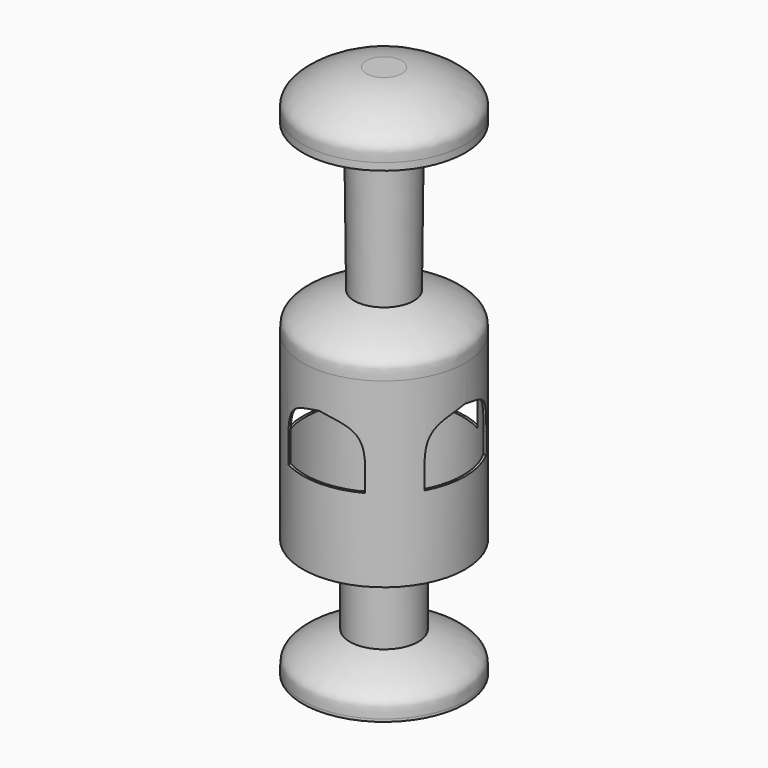
from build123d import *

# Parameters (mm, degrees)
F4_DEPTH = 25
F6_DEPTH = 25


# Not quite as in the source:
# - the dataset's text gives a spline's control points without its knots; the knots are read off the source's solid


with BuildPart() as f1:
    # F0 (on Front) → F1 (revolve)
    with BuildSketch(Plane.XZ):
        with BuildLine():
            Line((20.2840724203, -27.343348276), (23.0495763149, -27.3330021896))
            Line((23.0495763149, -27.3330021896), (23.0495763149, 24.1761978883))
            add(Edge.make_bspline(
                [(23.0495763149, 24.1761978883), (22.8941435237, 26.0308608144), (23.9395420726, 29.003648868), (14.0261189654, 33.6296849109), (8.4189805979, 34.9379997258)],
                knots=[0, 0, 0, 0, 0.3260886129, 0.8771804513, 0.8771804513, 0.8771804513, 0.8771804513], degree=3))
            add(Edge.make_bspline(
                [(8.4189805979, 34.9379997258), (8.1849872822, 34.992597437), (7.9520754508, 35.0444122094), (7.7206045906, 35.0932804837)],
                knots=[0.8771804513, 0.8771804513, 0.8771804513, 0.8771804513, 0.9001782441, 0.9001782441, 0.9001782441, 0.9001782441], degree=3))
            add(Edge.make_bspline(
                [(7.7206045906, 35.0932804837), (6.7159069707, 35.3053928798), (5.7383570717, 35.4619936087), (4.8173516989, 35.5497077107)],
                knots=[0.9001782441, 0.9001782441, 0.9001782441, 0.9001782441, 1, 1, 1, 1], degree=3))
            Line((4.8173516989, 35.5497077107), (0, 35.5497077107))
            Line((0, 35.5497077107), (0, 34.6961133182))
            Line((0, 34.6961133182), (4.8552267253, 34.6961133182))
            add(Edge.make_bspline(
                [(22.3495763149, 23.4555121765), (22.1897726726, 25.3623291907), (23.6752847702, 29.0289436305), (10.9884647614, 34.112000041), (4.8552267253, 34.6961133182)],
                knots=[0, 0, 0, 0, 0.3352583947, 1, 1, 1, 1], degree=3))
            Line((22.3495763149, 23.4555121765), (22.3495763149, -26.6947299242))
            Line((22.3495763149, -26.6947299242), (0, -26.6947299242))
            Line((0, -26.6947299242), (0, -27.4192334573))
            Line((0, -27.4192334573), (8.9649282769, -27.3856945706))
            Line((8.9649282769, -27.3856945706), (9.7, -27.3829445779))
            Line((9.7, -27.3829445779), (18.8340822147, -27.3487728656))
            Line((18.8340822147, -27.3487728656), (20.2840724203, -27.343348276))
        make_face()
    revolve(axis=Axis((0, 0, -7.0726890117), (0, 0, -1)))

    # F0 (on Front) → F2 (revolve)
    with BuildSketch(Plane.XZ):
        with BuildLine():
            add(Edge.make_bspline(
                [(23.0495763149, -60.2150011641), (22.8941435237, -58.3603382379), (23.8898585914, -55.5288345389), (14.9436544002, -51.1974927604), (9.7, -49.7765717533)],
                knots=[0, 0, 0, 0, 0.3260886129, 0.8354916825, 0.8354916825, 0.8354916825, 0.8354916825], degree=3))
            add(Edge.make_bspline(
                [(9.7, -49.7765717533), (9.4543795426, -49.7100137308), (9.2092217969, -49.6461323577), (8.9649282769, -49.5851103148)],
                knots=[0.8354916825, 0.8354916825, 0.8354916825, 0.8354916825, 0.8593528689, 0.8593528689, 0.8593528689, 0.8593528689], degree=3))
            add(Edge.make_bspline(
                [(8.9649282769, -49.5851103148), (7.5249670698, -49.2254226142), (6.1150323727, -48.9650789974), (4.8173516989, -48.8414913416)],
                knots=[0.8593528689, 0.8593528689, 0.8593528689, 0.8593528689, 1, 1, 1, 1], degree=3))
            Line((4.8173516989, -48.8414913416), (0, -48.8414913416))
            Line((0, -48.8414913416), (0, -49.6950857341))
            Line((0, -49.6950857341), (4.8552267253, -49.6950857341))
            add(Edge.make_bspline(
                [(22.3156850975, -60.2261610329), (22.2921596802, -58.7073440576), (23.1236631734, -55.1412446649), (10.9884647614, -50.2791990114), (4.8552267253, -49.6950857341)],
                knots=[0.0434798946, 0.0434798946, 0.0434798946, 0.0434798946, 0.3352583947, 1, 1, 1, 1], degree=3))
            add(Edge.make_bspline(
                [(22.3495763149, -60.9356868758), (22.3288512693, -60.6883904498), (22.3191907796, -60.4524902586), (22.3156850975, -60.2261610329)],
                knots=[0, 0, 0, 0, 0.0434798946, 0.0434798946, 0.0434798946, 0.0434798946], degree=3))
            Line((22.3495763149, -60.9356868758), (23.0495763149, -60.9422326088))
            Line((23.0495763149, -60.9422326088), (23.0495763149, -60.2150011641))
        make_face()
        with BuildLine():
            Line((9.7, -49.5851103148), (9.7, -27.3829445779))
            Line((9.7, -27.3829445779), (8.9649282769, -27.3856945706))
            Line((8.9649282769, -27.3856945706), (8.9649282769, -28.0694384128))
            Line((8.9649282769, -28.0694384128), (8.9649282769, -49.5851103148))
            add(Edge.make_bspline(
                [(9.7, -49.7765717533), (9.4543795426, -49.7100137308), (9.2092217969, -49.6461323577), (8.9649282769, -49.5851103148)],
                knots=[0.8354916825, 0.8354916825, 0.8354916825, 0.8354916825, 0.8593528689, 0.8593528689, 0.8593528689, 0.8593528689], degree=3))
            Line((9.7, -49.7765717533), (9.7, -49.5851103148))
        make_face()
        with BuildLine():
            Line((0, -60.9356868758), (22.3495763149, -60.9356868758))
            add(Edge.make_bspline(
                [(22.3495763149, -60.9356868758), (22.3288512693, -60.6883904498), (22.3191907796, -60.4524902586), (22.3156850975, -60.2261610329)],
                knots=[0, 0, 0, 0, 0.0434798946, 0.0434798946, 0.0434798946, 0.0434798946], degree=3))
            Line((22.3156850975, -60.2261610329), (0, -60.2261610329))
            Line((0, -60.2261610329), (0, -60.9356868758))
        make_face()
        Polygon((8.9649282769, -28.0694384128), (8.9649282769, -27.3856945706), (0, -27.4192334573), (0, -28.0694384128), align=None)
    revolve(axis=Axis((0, 0, -7.0726890117), (0, 0, -1)))

    # F3 (on Right) → F4 (cut, symmetric)
    with BuildSketch(Plane.YZ):
        with BuildLine():
            Line((-10.9680155292, -4.0999995545), (-0.0928910449, -4.0999995545))
            Line((-0.0928910449, -4.0999995545), (10.7822334394, -4.0999995545))
            Line((10.7822334394, -4.0999995545), (10.7822334394, 1.6936261673))
            add(Edge.make_bspline(
                [(10.7822334394, 1.6936261673), (10.8915483579, 10.6573491357), (8.377331309, 12.5156822614), (-0.0928910449, 14.0460734256)],
                knots=[0, 0, 0, 0, 16.4575601417, 16.4575601417, 16.4575601417, 16.4575601417], degree=3))
            add(Edge.make_bspline(
                [(-10.9680155292, 1.6936261673), (-11.0773304477, 10.6573491357), (-8.5631133988, 12.5156822614), (-0.0928910449, 14.0460734256)],
                knots=[0, 0, 0, 0, 16.4575601417, 16.4575601417, 16.4575601417, 16.4575601417], degree=3))
            Line((-10.9680155292, 1.6936261673), (-10.9680155292, -4.0999995545))
        make_face()
    extrude(amount=F4_DEPTH, both=True, mode=Mode.SUBTRACT)

    # F5 (on Front) → F6 (cut, symmetric)
    with BuildSketch(Plane.XZ):
        with BuildLine():
            Line((-10.8819976449, -3.9999997243), (-0.0068731606, -3.9999997243))
            Line((-0.0068731606, -3.9999997243), (10.8682513237, -3.9999997243))
            Line((10.8682513237, -3.9999997243), (10.8682513237, 1.7936259974))
            add(Edge.make_bspline(
                [(10.8682513237, 1.7936259974), (10.9775662422, 10.7573489659), (8.4633491933, 12.6156820916), (-0.0068731606, 14.1460732557)],
                knots=[0, 0, 0, 0, 16.4575601417, 16.4575601417, 16.4575601417, 16.4575601417], degree=3))
            add(Edge.make_bspline(
                [(-10.8819976449, 1.7936259974), (-10.9913125634, 10.7573489659), (-8.4770955145, 12.6156820916), (-0.0068731606, 14.1460732557)],
                knots=[0, 0, 0, 0, 16.4575601417, 16.4575601417, 16.4575601417, 16.4575601417], degree=3))
            Line((-10.8819976449, 1.7936259974), (-10.8819976449, -3.9999997243))
        make_face()
    extrude(amount=F6_DEPTH, both=True, mode=Mode.SUBTRACT)

    # F0 (on Front) → F7 (revolve)
    with BuildSketch(Plane.XZ):
        with BuildLine():
            add(Edge.make_bspline(
                [(8.4189805979, 34.9379997258), (8.1849872822, 34.992597437), (7.9520754508, 35.0444122094), (7.7206045906, 35.0932804837)],
                knots=[0.8771804513, 0.8771804513, 0.8771804513, 0.8771804513, 0.9001782441, 0.9001782441, 0.9001782441, 0.9001782441], degree=3))
            Line((8.4189805979, 34.9379997258), (8.865498937, 76.6738313739))
            Line((8.865498937, 76.6738313739), (23.0495763148, 76.6738313739))
            Line((23.0495763148, 76.6738313739), (23.0495763148, 78.7230981444))
            add(Edge.make_bspline(
                [(23.0495763148, 78.7230981444), (23.0495763148, 80.6078122564), (23.9507031304, 83.9578134153), (11.2077367667, 90.5497077107), (5, 90.5497077107)],
                knots=[0, 0, 0, 0, 0.3302146344, 1, 1, 1, 1], degree=3))
            Line((5, 90.5497077107), (0, 90.5497077107))
            Line((0, 90.5497077107), (0, 89.8497104645))
            Line((0, 89.8497104645), (5, 89.8497104645))
            add(Edge.make_bspline(
                [(22.3495790686, 78.7230981444), (22.3495790686, 79.0937647853), (22.3716877562, 79.7678791576), (22.3933148354, 80.6007538754), (22.3399061529, 81.2821155275), (22.1725915882, 81.8776125403), (21.8790408964, 82.4045882825), (21.4922195357, 82.886710278), (20.9908563885, 83.4132154485), (20.1707115884, 84.1274223788), (18.9256521099, 85.0269281278), (17.4668159276, 85.9325369699), (15.2961373534, 87.1052139435), (12.269445396, 88.4292040949), (8.4841313235, 89.5564062965), (6.0965880095, 89.8497104645), (5, 89.8497104645)],
                knots=[0, 0, 0, 0, 0.0625, 0.125, 0.1875, 0.25, 0.3125, 0.34375, 0.375, 0.4375, 0.5, 0.5625, 0.625, 0.75, 0.875, 1, 1, 1, 1], degree=3))
            Line((22.3495790686, 78.7230981444), (22.3495790686, 77.3738286202))
            Line((22.3495790686, 77.3738286202), (8.1729506775, 77.3738286202))
            Line((8.1729506775, 77.3738286202), (7.7206045906, 35.0932804837))
        make_face()
    revolve(axis=Axis((0, 0, 62.5293496996), (0, 0, -1)))


solid = f1.part
